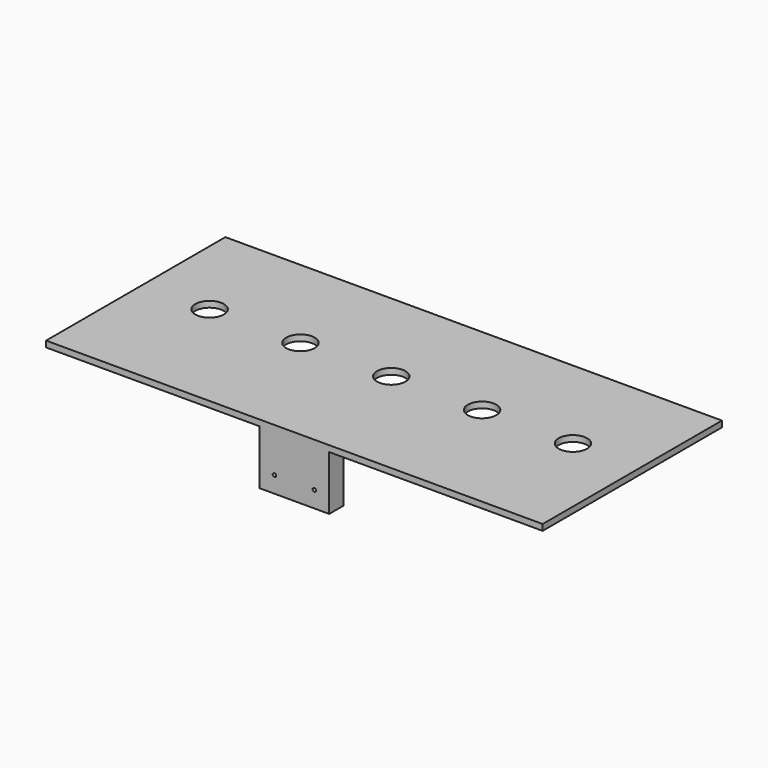
from build123d import *

# Parameters (mm, degrees)
F0_W          = 208.28
F0_H          = 93.98
F1_DEPTH      = 2.54
F2_R          = 5.969
F3_DEPTH      = 2.541
F4_DEPTH      = 6.604
F2_W          = 29.21
F2_H          = 7.62
F5_DEPTH      = 25.4
F7_D          = 1.016
F7_DEPTH      = 10.16
F7_TIP        = 0.3052371945
F9_D          = 1.4732
F9_DEPTH      = 10.16
F9_TIP        = 0.442593932
F10_TEXT_SIZE = 26.2611700843
F11_DEPTH     = 1.524


# Not quite as in the source:
# - a feature names something its author has since deleted; it is built from what else it names
# - Text() gives the source's letters only with a copy of the font that has no kerning and outlines rounded to 1/6400 em; it was checked with that copy


with BuildPart() as f1:
    # F0 (on Top) → F1 (new body)
    with BuildSketch(Plane.XY):
        Rectangle(F0_W, F0_H)
    extrude(amount=F1_DEPTH)

    # F2 (on face) → F3 (cut, through all)
    with BuildSketch(Plane.XY.offset(2.54)):
        with Locations((-76.2, 3.81)):
            Circle(F2_R)
        with Locations((-38.1, 3.81)):
            Circle(F2_R)
        with Locations((38.1, 3.81)):
            Circle(F2_R)
        with Locations((76.2, 3.81)):
            Circle(F2_R)
        Polygon((-50.8, 46.99), (-41.021, 46.99), (-41.021, 59.69), (-60.579, 59.69), (-60.579, 46.99), align=None)
        Polygon((41.021, 59.69), (41.021, 46.99), (50.8, 46.99), (60.579, 46.99), (60.579, 59.69), align=None)
        with Locations((0, 3.81)):
            Circle(F2_R)
    extrude(amount=-F3_DEPTH, mode=Mode.SUBTRACT)

    # F2 (on face) → F4 (join)
    with BuildSketch(Plane.XY.offset(2.54)):
        Polygon((-41.021, 34.29), (-41.021, 46.99), (-50.8, 46.99), (-60.579, 46.99), (-60.579, 34.29), align=None)
        Polygon((50.8, 46.99), (41.021, 46.99), (41.021, 34.29), (60.579, 34.29), (60.579, 46.99), align=None)
    extrude(amount=-F4_DEPTH)

    # F2 (on face) → F5 (join)
    with BuildSketch(Plane.XY.offset(2.54)):
        with Locations((0, -43.18)):
            Rectangle(F2_W, F2_H)
    extrude(amount=-F5_DEPTH)

    # F7
    with Locations(Plane(origin=(0, 46.99, 0), x_dir=(-1, 0, 0), z_dir=(0, 1, 0))):
        with Locations((-56.3118, -1.016), (-45.2882, -1.016), (45.2882, -1.016), (56.3118, -1.016)):
            Hole(F7_D / 2, depth=F7_DEPTH)
            with Locations((0, 0, -(F7_DEPTH + F7_TIP / 2))):  # 118° drill point
                Cone(0, F7_D / 2, F7_TIP, mode=Mode.SUBTRACT)

    # F9
    with Locations(Plane.XZ.offset(46.99)):
        with Locations((8.3566, -16.002), (-8.3566, -16.002)):
            Hole(F9_D / 2, depth=F9_DEPTH)
            with Locations((0, 0, -(F9_DEPTH + F9_TIP / 2))):  # 118° drill point
                Cone(0, F9_D / 2, F9_TIP, mode=Mode.SUBTRACT)

    # F10 (on face) → F11 (join)
    with BuildSketch(Plane(origin=(0, 0, 0), x_dir=(1, 0, 0), z_dir=(0, 0, -1))):
        with Locations((-70.6348344684, 18.5782536864)):
            Text('BOOM BOX', F10_TEXT_SIZE, font='Open Sans', text_align=(TextAlign.LEFT, TextAlign.BOTTOM))
    extrude(amount=F11_DEPTH)


solid = f1.part
